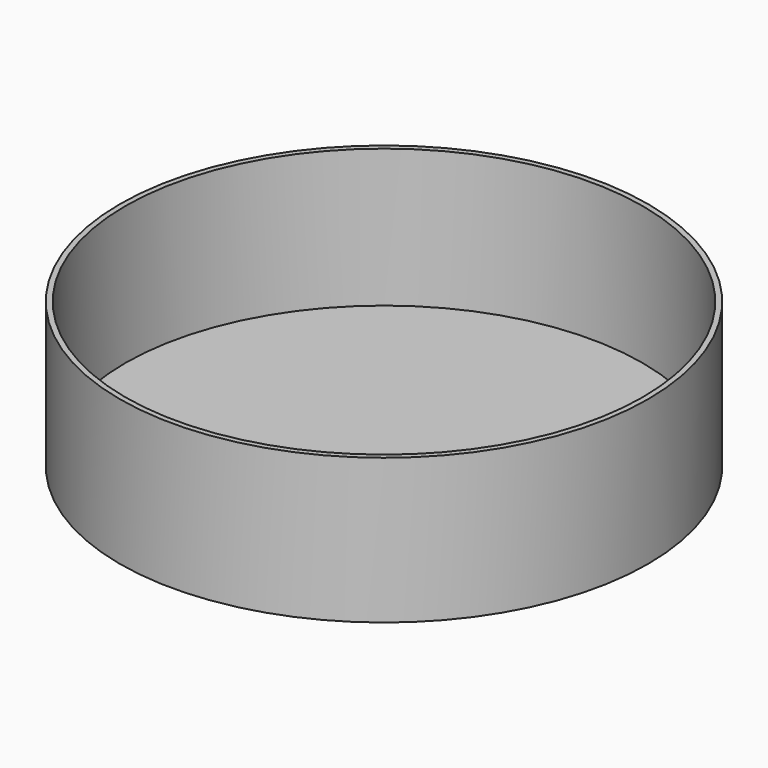
from build123d import *

# Parameters (mm, degrees)
F0_R     = 75
F1_DEPTH = 2
F2_W     = 1.5584379435
F2_H     = 42.0504882932


# Not quite as in the source:
# - a feature names something its author has since deleted; it is built from what else it names


with BuildPart() as f1:
    # F0 (on Top) → F1 (new body)
    with BuildSketch(Plane.XY):
        Circle(F0_R)
    extrude(amount=F1_DEPTH)


with BuildPart() as f3:
    # F2 (on Front) → F3 (revolve)
    with BuildSketch(Plane.XZ):
        with Locations((75.7932811975, 21.0252441466)):
            Rectangle(F2_W, F2_H)
    revolve(axis=Axis((0, 0, 2), (0, 0, 1)))


solid = Compound([f1.part, f3.part])
